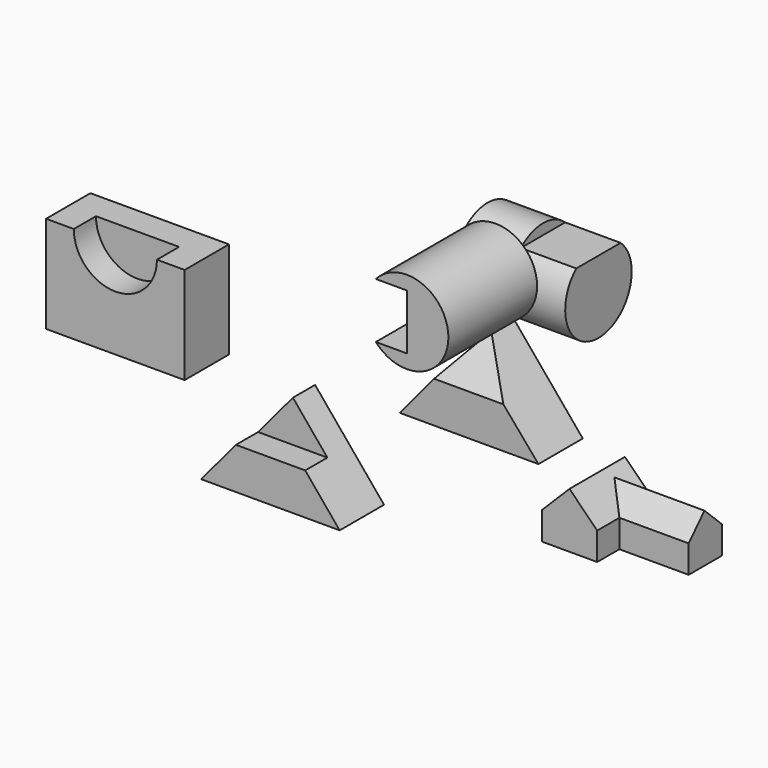
from build123d import *

# Parameters (mm, degrees)
F1_DEPTH  = 101.6
F3_DEPTH  = 50.8
F5_DEPTH  = 254
F7_DEPTH  = 254
F9_DEPTH  = 254
F11_DEPTH = 127
F12_W     = 76.2
F12_H     = 50.8
F13_DEPTH = 127
F15_R     = 76.2
F16_DEPTH = 203.2
F18_DEPTH = 101.6
F19_R     = 76.2
F20_DEPTH = 203.2
F22_DEPTH = 101.6
F23_W     = 254
F23_H     = 177.8
F24_DEPTH = 101.6
F26_DEPTH = 50.8


with BuildPart() as f1:
    # F0 (on Front) → F1 (new body)
    with BuildSketch(Plane.XZ):
        Polygon((0, 0), (-127.6350005588, -152.4), (126.3649994412, -152.4), align=None)
    extrude(amount=F1_DEPTH)

    # F2 (on face) → F3 (cut)
    with BuildSketch(Plane.XZ.offset(101.6)):
        Polygon((0, 0), (-63.8175002794, -76.2), (63.1824997206, -76.2), align=None)
    extrude(amount=-F3_DEPTH, mode=Mode.SUBTRACT)


with BuildPart() as f5:
    # F4 (on Right) → F5 (new body)
    with BuildSketch(Plane.YZ):
        Polygon((193.3565672969, -48.0408182748), (194.32102892, -124.2347144462), (295.92102892, -124.2347144462), (295.92102892, 28.1652855538), (245.12102892, 28.1652855538), align=None)
    extrude(amount=F5_DEPTH)

    # F6 (on face) → F7 (cut)
    with BuildSketch(Plane(origin=(0, 295.92102892, 0), x_dir=(-1, 0, 0), z_dir=(0, 1, 0))):
        Polygon((-254, 28.1652855538), (-254, -124.2347144462), (-127, 28.1652855538), align=None)
    extrude(amount=-F7_DEPTH, mode=Mode.SUBTRACT)

    # F8 (on face) → F9 (cut)
    with BuildSketch(Plane(origin=(0, 295.92102892, 0), x_dir=(-1, 0, 0), z_dir=(0, 1, 0))):
        Polygon((-127, 28.1652855538), (0, -124.2347144462), (0, 28.1652855538), align=None)
    extrude(amount=-F9_DEPTH, mode=Mode.SUBTRACT)


with BuildPart() as f11:
    # F10 (on Front) → F11 (new body)
    with BuildSketch(Plane.XZ):
        Polygon((415.6096123431, -66.908387676), (415.6096123431, -117.708387676), (517.2096123431, -117.708387676), (517.2096123431, -66.908387676), (466.4096123431, -16.108387676), align=None)
    extrude(amount=-F11_DEPTH)

    # F12 (on face) → F13 (join)
    with BuildSketch(Plane.YZ.offset(517.2096123431)):
        with Locations((88.9, -92.308387676)):
            Rectangle(F12_W, F12_H)
        Polygon((50.8, -66.908387676), (127, -66.908387676), (86.994998771, -28.808387676), align=None)
    extrude(amount=F13_DEPTH)

    # F12 (on face) → F14 (join, up to the next surface of F11)
    with BuildSketch(Plane.YZ.offset(517.2096123431)):
        Polygon((50.8, -66.908387676), (127, -66.908387676), (86.994998771, -28.808387676), align=None)
    extrude(until=Until.NEXT, dir=(-1, 0, 0))


with BuildPart() as f16:
    # F15 (on Right) → F16 (new body)
    with BuildSketch(Plane.YZ):
        with Locations((395.3134715557, 57.1514479816)):
            Circle(F15_R)
    extrude(amount=F16_DEPTH)

    # F17 (on face) → F18 (cut)
    with BuildSketch(Plane.YZ.offset(203.2)):
        with BuildLine():
            ThreePointArc((446.1134715557, 113.9475746101), (395.3134715557, 133.3514479816), (344.5134715557, 113.9475746101))
            Line((344.5134715557, 113.9475746101), (446.1134715557, 113.9475746101))
        make_face()
    extrude(amount=-F18_DEPTH, mode=Mode.SUBTRACT)


with BuildPart() as f20:
    # F19 (on Front) → F20 (new body)
    with BuildSketch(Plane.XZ):
        with Locations((330.7407200336, 291.7511761189)):
            Circle(F19_R)
    extrude(amount=F20_DEPTH)

    # F21 (on face) → F22 (cut)
    with BuildSketch(Plane.XZ.offset(203.2)):
        with BuildLine():
            Line((330.7407200336, 342.5511761189), (273.9445934052, 342.5511761189))
            ThreePointArc((273.9445934052, 342.5511761189), (254.5407200336, 291.7511761189), (273.9445934052, 240.9511761189))
            Line((273.9445934052, 240.9511761189), (330.7407200336, 240.9511761189))
            Line((330.7407200336, 240.9511761189), (330.7407200336, 342.5511761189))
        make_face()
    extrude(amount=-F22_DEPTH, mode=Mode.SUBTRACT)


with BuildPart() as f24:
    # F23 (on Front) → F24 (new body)
    with BuildSketch(Plane.XZ):
        with Locations((-284.8508283496, 86.5570213336)):
            Rectangle(F23_W, F23_H)
    extrude(amount=F24_DEPTH)

    # F25 (on face) → F26 (cut)
    with BuildSketch(Plane.XZ.offset(101.6)):
        with BuildLine():
            Line((-361.0508283496, 175.4570213336), (-208.6508283496, 175.4570213336))
            ThreePointArc((-208.6508283496, 175.4570213336), (-284.8508283496, 251.6570213336), (-361.0508283496, 175.4570213336))
        make_face()
        with BuildLine():
            ThreePointArc((-361.0508283496, 175.4570213336), (-284.8508283496, 99.2570213336), (-208.6508283496, 175.4570213336))
            Line((-208.6508283496, 175.4570213336), (-361.0508283496, 175.4570213336))
        make_face()
    extrude(amount=-F26_DEPTH, mode=Mode.SUBTRACT)


solid = Compound([f1.part, f5.part, f11.part, f16.part, f20.part, f24.part])
